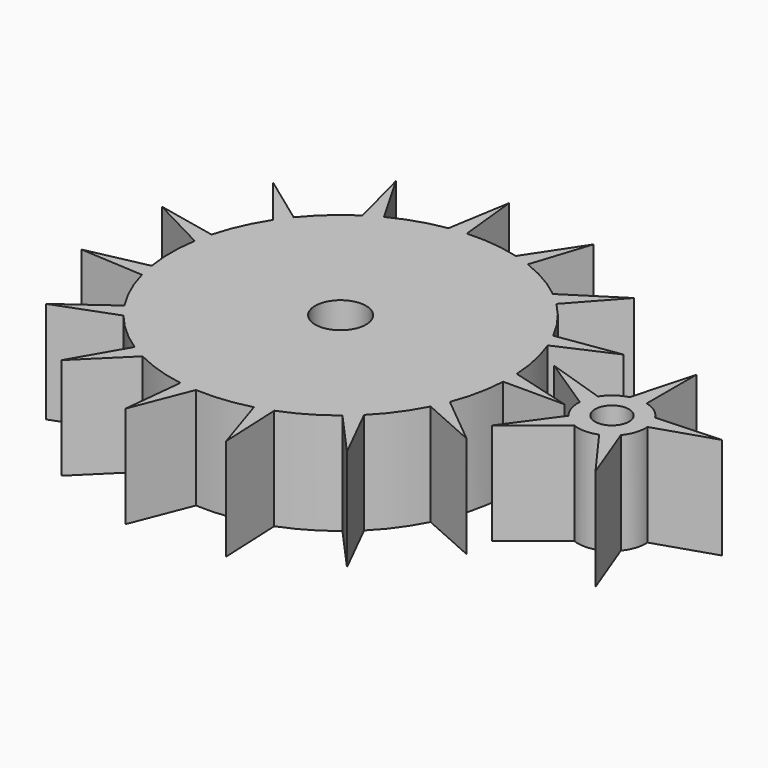
from build123d import *

# Parameters (mm, degrees)
F0_R            = 63.5
F1_DEPTH        = 38.1
F0_R_2          = 12.7
F3_DEPTH        = 38.1
F3_COPIES_COUNT = 15
F6_DEPTH        = 38.1
F6_COPIES_COUNT = 5
F7_R            = 9.525
F7_R_2          = 6.35
F8_DEPTH        = 38.101


# Not quite as in the source:
# - a pattern or mirror of a feature is missing from the dataset's text; its kind, count and spacing are read off the source's solid


with BuildPart() as f1:
    # F0 (on Top) → F1 (new body)
    with BuildSketch(Plane.XY):
        with Locations((-77.2365369129, 0)):
            Circle(F0_R)
    extrude(amount=F1_DEPTH)

    # F2 (on face) → F3 (join)
    with BuildSketch(Plane.XY.offset(38.1)):
        Polygon((-13.8159615844, 3.175), (-77.2365369129, 3.175), (-77.2365369129, -3.175), (9.1234630871, -3.175), align=None)
    f3 = extrude(amount=-F3_DEPTH)

    # F3_copies: F3 ×15 about axis
    f3_copies_axis = Axis((-77.236537, 0, 0), (0, 0, 1))
    for i in range(1, F3_COPIES_COUNT):
        add(f3.rotate(f3_copies_axis, i * 360 / F3_COPIES_COUNT))


with BuildPart() as f1b:
    # F0 (on Top) → F1, piece 2 (new body)
    with BuildSketch(Plane.XY):
        with Locations((24.3634630871, 0)):
            Circle(F0_R_2)
    extrude(amount=F1_DEPTH)

    # F5 (on face) → F6 (join)
    with BuildSketch(Plane.XY.offset(38.1)):
        Polygon((21.1884630871, 0), (27.5384630871, 0), (27.5384630871, 35.56), (21.1884630871, 12.2967221242), align=None)
    f6 = extrude(amount=-F6_DEPTH)

    # F6_copies: F6 ×5 about axis
    f6_copies_axis = Axis((24.363463, 0, 0), (0, 0, 1))
    for i in range(1, F6_COPIES_COUNT):
        add(f6.rotate(f6_copies_axis, i * 360 / F6_COPIES_COUNT))


with BuildPart() as f8_tool:
    # F7 (on face) → F8 (new body, through all)
    with BuildSketch(Plane.XY.offset(38.1)):
        with Locations((-77.2365369129, 0)):
            Circle(F7_R)
        with Locations((24.3634630871, 0)):
            Circle(F7_R_2)
    extrude(amount=-F8_DEPTH)


with BuildPart() as f1_1:
    add(f1.part)

    # F8: cut by f8_tool
    add(f8_tool.part, mode=Mode.SUBTRACT)


with BuildPart() as f1b_1:
    add(f1b.part)

    # F8: cut by f8_tool
    add(f8_tool.part, mode=Mode.SUBTRACT)


solid = Compound([f1_1.part, f1b_1.part])
